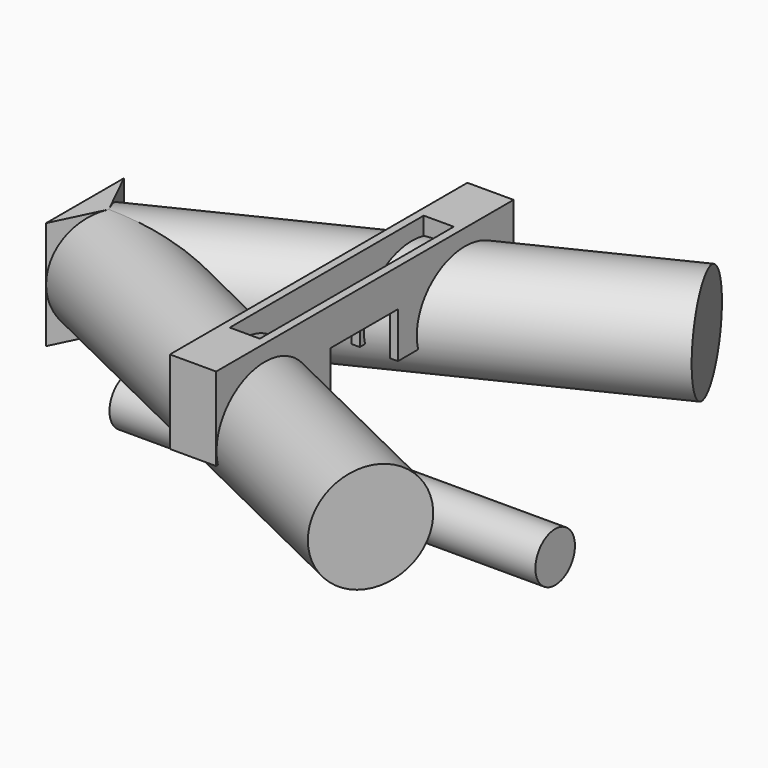
from build123d import *

# Parameters (mm, degrees)
F3_DEPTH = 16.75
F4_W     = 14.3
F4_H     = 115
F4_W_2   = 9.3
F4_H_2   = 75
F5_DEPTH = 20.75
F6_DEPTH = 5
F7_W     = 26.0475566859
F7_H     = 14.153759297
F8_DEPTH = 25
F9_W     = 131.7364319801
F9_H     = 7.65


# Not quite as in the source:
# - a feature of the source that left no trace in its solid (it failed there, or was rolled back) is left out


with BuildPart() as f1:
    # F0 (on Top) → F1 (revolve)
    with BuildSketch(Plane.XY):
        Polygon((-134.3117827935, 15.0481095387), (-126.9553638746, 0), (-50.2462865474, 37.5), (6.0070368258, 65), (-1.3493820931, 80.0481095387), align=None)
    revolve(axis=Axis((-60.4741635244, 32.5, 0), (0.8983945993, 0.4391891892, 0)))

    # F0 (on Top) → F2 (revolve)
    with BuildSketch(Plane.XY):
        Polygon((-50.2462865474, -37.5), (-126.9553638746, 0), (-134.3117827935, -15.0481095387), (-1.3493820931, -80.0481095387), (6.0070368258, -65), align=None)
    revolve(axis=Axis((-60.4741635244, -32.5, 0), (-0.8983945993, 0.4391891892, 0)))

    # F0 (on Top) → F3 (join, symmetric)
    with BuildSketch(Plane.XY):
        Polygon((-134.3117827935, -15.0481095387), (-126.9553638746, 0), (-134.3117827935, 15.0481095387), align=None)
    extrude(amount=F3_DEPTH, both=True)


with BuildPart() as f5:
    # F4 (on face) → F5 (new body)
    with BuildSketch(Plane.XY.offset(16.75)):
        with Locations((-54.8962865474, 0)):
            Rectangle(F4_W, F4_H)
        with Locations((-54.8962865474, 0)):
            Rectangle(F4_W_2, F4_H_2, mode=Mode.SUBTRACT)
    extrude(amount=-F5_DEPTH)

    # F4 (on face) → F6 (join)
    with BuildSketch(Plane.XY.offset(16.75)):
        with Locations((-54.8962865474, 0)):
            Rectangle(F4_W, F4_H)
        with Locations((-54.8962865474, 0)):
            Rectangle(F4_W_2, F4_H_2, mode=Mode.SUBTRACT)
    extrude(amount=F6_DEPTH)

    # F7 (on face) → F8 (cut)
    with BuildSketch(Plane(origin=(-62.0462865474, 0, 0), x_dir=(0, -1, 0), z_dir=(-1, 0, 0))):
        with Locations((0.2447417813, 3.0768796485)):
            Rectangle(F7_W, F7_H)
    extrude(amount=-F8_DEPTH, mode=Mode.SUBTRACT)


with BuildPart() as f10:
    # F9 (on Front) → F10 (revolve)
    with BuildSketch(Plane.XZ):
        with Locations((-54.7559685074, -29.175)):
            Rectangle(F9_W, F9_H)
    revolve(axis=Axis((-54.7559685074, 0, -33), (1, 0, 0)))


solid = Compound([f1.part, f5.part, f10.part])
